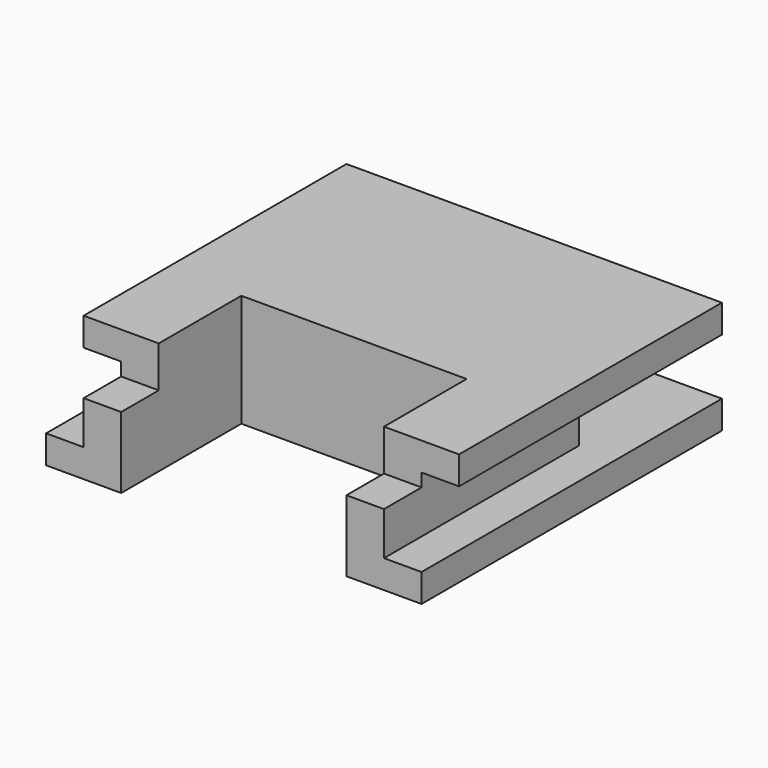
from build123d import *

# Parameters (mm, degrees)
F1_DEPTH = 1.5
F3_DEPTH = 3
F5_DEPTH = 1.5
F6_W     = 4
F6_H     = 2.5
F7_DEPTH = 2.2


# Not quite as in the source:
# - a feature names something its author has since deleted; it is built from what else it names


with BuildPart() as f1:
    # F0 (on Top) → F1 (new body)
    with BuildSketch(Plane.XY):
        Polygon((10, 12), (-10, 12), (-10, -8), (-6, -8), (-6, 0), (6, 0), (6, -8), (10, -8), align=None)
    extrude(amount=F1_DEPTH)

    # F2 (on face) → F3 (join)
    with BuildSketch(Plane.XY.offset(1.5)):
        Polygon((-8, 5), (-8, -8), (-6, -8), (-6, 0), (6, 0), (6, -8), (8, -8), (8, 5), align=None)
    extrude(amount=F3_DEPTH)

    # F4 (on face) → F5 (join)
    with BuildSketch(Plane.XY.offset(4.5)):
        Polygon((-8, -8), (-6, -8), (-6, 0), (6, 0), (6, -8), (8, -8), (8, 5), (-8, 5), align=None)
        Polygon((-10, -8), (-8, -8), (-8, 5), (8, 5), (8, -8), (10, -8), (10, 12), (-10, 12), align=None)
    extrude(amount=F5_DEPTH)

    # F6 (on face) → F7 (cut)
    with BuildSketch(Plane.XY.offset(6)):
        with Locations((-8, -6.75)):
            Rectangle(F6_W, F6_H)
        with Locations((8, -6.75)):
            Rectangle(F6_W, F6_H)
    extrude(amount=-F7_DEPTH, mode=Mode.SUBTRACT)


solid = f1.part
